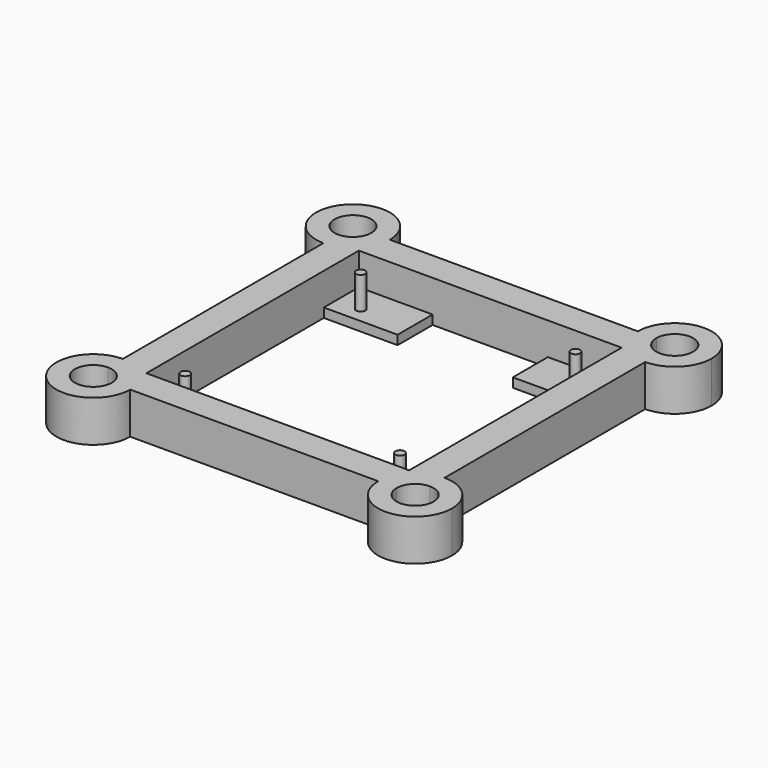
from build123d import *

# Parameters (mm, degrees)
F1_DEPTH = 4.5
F0_R     = 0.5
F2_W     = 28.5
F2_H     = 4.75
F2_H_2   = 4.77
F3_DEPTH = 1
F5_W     = 12.5
F5_H     = 4.75
F5_W_2   = 16.5
F5_H_2   = 4.77
F6_DEPTH = 3.5


with BuildPart() as f1:
    # F0 (on Top) → F1 (new body)
    with BuildSketch(Plane.XY):
        with BuildLine():
            Line((17.45, -13.6), (17.45, 13.6))
            ThreePointArc((17.45, 13.6), (14.6215728753, 14.7715728753), (13.45, 17.6))
            Line((13.45, 17.6), (-13.45, 17.6))
            ThreePointArc((-13.45, 17.6), (-14.6215728753, 14.7715728753), (-17.45, 13.6))
            Line((-17.45, 13.6), (-17.45, -13.6))
            ThreePointArc((-17.45, -13.6), (-14.6215728753, -14.7715728753), (-13.45, -17.6))
            Line((-13.45, -17.6), (13.45, -17.6))
            ThreePointArc((13.45, -17.6), (14.6215728753, -14.7715728753), (17.45, -13.6))
        make_face()
        Polygon((-14.25, 9.65), (-14.25, 14.4), (14.25, 14.4), (14.25, 9.65), (14.25, -9.63), (14.25, -14.4), (-14.25, -14.4), (-14.25, -9.63), align=None, mode=Mode.SUBTRACT)
        with BuildLine():
            Line((-15.45, 17.6), (-13.45, 17.6))
            ThreePointArc((-13.45, 17.6), (-20.2784271247, 20.4284271247), (-17.45, 13.6))
            Line((-17.45, 13.6), (-17.45, 15.6))
            ThreePointArc((-17.45, 15.6), (-18.8642135624, 19.0142135624), (-15.45, 17.6))
        make_face()
        with BuildLine():
            ThreePointArc((19.45, 17.6), (18.8642135624, 16.1857864376), (17.45, 15.6))
            Line((17.45, 15.6), (17.45, 13.6))
            ThreePointArc((17.45, 13.6), (20.2784271247, 14.7715728753), (21.45, 17.6))
            ThreePointArc((21.45, 17.6), (17.45, 21.6), (13.45, 17.6))
            Line((13.45, 17.6), (15.45, 17.6))
            ThreePointArc((15.45, 17.6), (17.45, 19.6), (19.45, 17.6))
        make_face()
        with BuildLine():
            ThreePointArc((21.45, -17.6), (20.2784271247, -14.7715728753), (17.45, -13.6))
            Line((17.45, -13.6), (17.45, -15.6))
            ThreePointArc((17.45, -15.6), (18.8642135624, -16.1857864376), (19.45, -17.6))
            ThreePointArc((19.45, -17.6), (17.45, -19.6), (15.45, -17.6))
            Line((15.45, -17.6), (13.45, -17.6))
            ThreePointArc((13.45, -17.6), (17.45, -21.6), (21.45, -17.6))
        make_face()
        with BuildLine():
            ThreePointArc((-17.45, -13.6), (-20.2784271247, -20.4284271247), (-13.45, -17.6))
            Line((-13.45, -17.6), (-15.45, -17.6))
            ThreePointArc((-15.45, -17.6), (-18.8642135624, -19.0142135624), (-17.45, -15.6))
            Line((-17.45, -15.6), (-17.45, -13.6))
        make_face()
        with BuildLine():
            ThreePointArc((-17.45, 13.6), (-14.6215728753, 14.7715728753), (-13.45, 17.6))
            Line((-13.45, 17.6), (-15.45, 17.6))
            ThreePointArc((-15.45, 17.6), (-16.0357864376, 16.1857864376), (-17.45, 15.6))
            Line((-17.45, 15.6), (-17.45, 13.6))
        make_face()
        with BuildLine():
            Line((17.45, 13.6), (17.45, 15.6))
            ThreePointArc((17.45, 15.6), (16.0357864376, 16.1857864376), (15.45, 17.6))
            Line((15.45, 17.6), (13.45, 17.6))
            ThreePointArc((13.45, 17.6), (14.6215728753, 14.7715728753), (17.45, 13.6))
        make_face()
        with BuildLine():
            Line((17.45, -15.6), (17.45, -13.6))
            ThreePointArc((17.45, -13.6), (14.6215728753, -14.7715728753), (13.45, -17.6))
            Line((13.45, -17.6), (15.45, -17.6))
            ThreePointArc((15.45, -17.6), (16.0357864376, -16.1857864376), (17.45, -15.6))
        make_face()
        with BuildLine():
            Line((-15.45, -17.6), (-13.45, -17.6))
            ThreePointArc((-13.45, -17.6), (-14.6215728753, -14.7715728753), (-17.45, -13.6))
            Line((-17.45, -13.6), (-17.45, -15.6))
            ThreePointArc((-17.45, -15.6), (-16.0357864376, -16.1857864376), (-15.45, -17.6))
        make_face()
    extrude(amount=F1_DEPTH)

    # F2 (on Top) → F3 (join)
    with BuildSketch(Plane.XY):
        with Locations((0, 12.025)):
            Rectangle(F2_W, F2_H)
        with Locations((0, -12.015)):
            Rectangle(F2_W, F2_H_2)
    extrude(amount=F3_DEPTH)

    # F5 (on offset) → F6 (cut)
    with BuildSketch(Plane.XY.offset(3.5)):
        with Locations((0, 12.025)):
            Rectangle(F5_W, F5_H)
        with Locations((0, -12.015)):
            Rectangle(F5_W_2, F5_H_2)
    extrude(amount=-F6_DEPTH, mode=Mode.SUBTRACT)


with BuildPart() as f1b:
    # F0 (on Top) → F1, piece 2 (new body)
    with BuildSketch(Plane.XY):
        with Locations((-11.65, 11.4)):
            Circle(F0_R)
    extrude(amount=F1_DEPTH)


with BuildPart() as f1c:
    # F0 (on Top) → F1, piece 3 (new body)
    with BuildSketch(Plane.XY):
        with Locations((11.65, 11.4)):
            Circle(F0_R)
    extrude(amount=F1_DEPTH)


with BuildPart() as f1d:
    # F0 (on Top) → F1, piece 4 (new body)
    with BuildSketch(Plane.XY):
        with Locations((11.65, -12.4)):
            Circle(F0_R)
    extrude(amount=F1_DEPTH)


with BuildPart() as f1e:
    # F0 (on Top) → F1, piece 5 (new body)
    with BuildSketch(Plane.XY):
        with Locations((-11.65, -12.4)):
            Circle(F0_R)
    extrude(amount=F1_DEPTH)


solid = Compound([f1.part, f1b.part, f1c.part, f1d.part, f1e.part])
